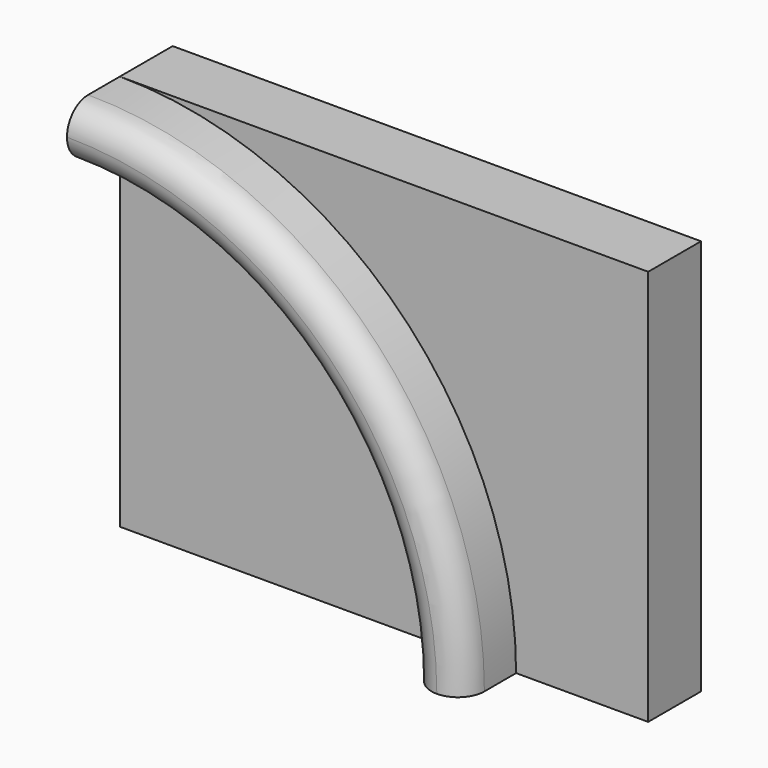
from build123d import *

# Parameters (mm, degrees)
F0_W     = 101.6
F0_H     = 76.2
F1_DEPTH = 12.7
F3_DEPTH = 25.4
F4_R     = 5.07999


# Not quite as in the source:
# - a fillet or chamfer is up to 0.001 mm smaller than in the source, because OpenCascade refuses the exact size


with BuildPart() as f1:
    # F0 (on Front) → F1 (new body)
    with BuildSketch(Plane.XZ):
        with Locations((50.8, 38.1)):
            Rectangle(F0_W, F0_H)
    extrude(amount=F1_DEPTH)


with BuildPart() as f3:
    # F2 (on Front) → F3 (new body)
    with BuildSketch(Plane.XZ):
        with BuildLine():
            ThreePointArc((76.2, 0), (53.8815367264, 53.8815367264), (0, 76.2))
            Line((0, 76.2), (0, 66.04))
            ThreePointArc((0, 66.04), (46.6973318296, 46.6973318296), (66.04, 0))
            Line((66.04, 0), (76.2, 0))
        make_face()
    extrude(amount=F3_DEPTH)

    # F4 (radius 5.08 in the source; OpenCascade refuses exactly that, so slightly less here)
    f4_edges = [f3.edges().sort_by_distance(p)[0] for p in [
        (46.697332, -25.4, 46.697332),
        (53.881537, -25.4, 53.881537),
    ]]
    fillet(f4_edges, radius=F4_R)


solid = Compound([f1.part, f3.part])
